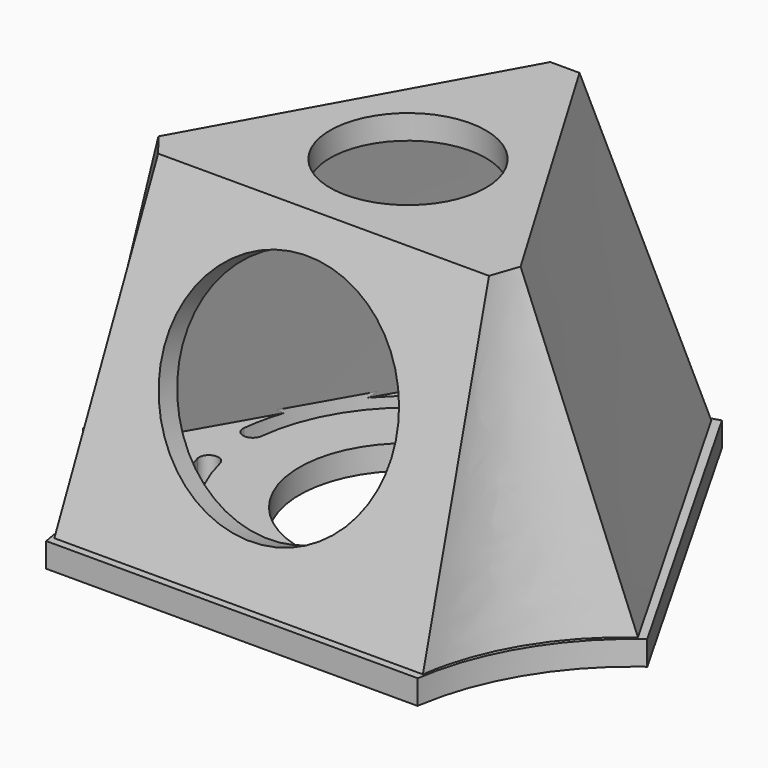
from build123d import *

# Parameters (mm, degrees)
F4_T      = -2.5
F6_R      = 8
F7_DEPTH  = 2.5
F9_DEPTH  = 2.5
F5_R      = 11.15
F10_DEPTH = 2.5
F12_DEPTH = 3
F14_R     = 12
F15_DEPTH = 2.5


with BuildPart() as f3:
    # F1 (on Top) → F3 section 0
    with BuildSketch(Plane.XY):
        with BuildLine():
            Line((-9.9467867985, 28.3880904317), (-28.9289951324, -4.7229221091))
            ThreePointArc((-28.9289951324, -4.7229221091), (-22.2240470788, -12.2883453364), (-19.0064776689, -21.8716226518))
            Line((-19.0064776689, -21.8716226518), (19.1736482084, -21.8716226518))
            ThreePointArc((19.1736482084, -21.8716226518), (22.5091585374, -12.4144453799), (29.3118748814, -5.0464821979))
            Line((29.3118748814, -5.0464821979), (10.2218100801, 28.3880904317))
            ThreePointArc((10.2218100801, 28.3880904317), (0.1375116408, 26.6367572465), (-9.9467867985, 28.3880904317))
        make_face()
    # F2 (on offset) → F3 section 1
    with BuildSketch(Plane.XY.offset(34)):
        Polygon((-1.6149276096, 21.1612877117), (-18.1069700896, -8.5710605783), (-16.2452941719, -10.9235407117), (17.7547058281, -10.9235407117), (18.7248919411, -8.0847489077), (1.3850723904, 21.1612877117), align=None)
    loft()

    # F4
    f4_openings = [f3.faces().sort_by_distance(p)[0] for p in [
        (0.146214, 0.67534, 0),
    ]]
    offset(amount=F4_T, openings=f4_openings)

    # F6 (on offset) → F7 (cut, through all)
    with BuildSketch(Plane.XY.offset(34)):
        with Locations((0, 0.8572275097)):
            Circle(F6_R)
    extrude(amount=-F7_DEPTH, mode=Mode.SUBTRACT)

    # F8 (on Top) → F9 (join)
    with BuildSketch(Plane.XY):
        with BuildLine():
            Line((-9.9509973079, 28.3981114626), (-28.9402902126, -4.7158375382))
            ThreePointArc((-28.9402902126, -4.7158375382), (-22.262978648, -12.2971961913), (-18.9997616398, -21.8583103269))
            Line((-18.9997616398, -21.8583103269), (19.1731229424, -21.8583103269))
            ThreePointArc((19.1731229424, -21.8583103269), (22.5411210843, -12.4278954037), (29.305677861, -5.044338759))
            Line((29.305677861, -5.044338759), (10.2393915877, 28.3862594515))
            ThreePointArc((10.2393915877, 28.3862594515), (0.1431471721, 26.6035220267), (-9.9509973079, 28.3981114626))
        make_face()
    extrude(amount=F9_DEPTH)

    # F5 (on Top) → F10 (cut, through all)
    with BuildSketch(Plane.XY):
        with Locations((0, 0.8448960521)):
            Circle(F5_R)
    extrude(amount=F10_DEPTH, mode=Mode.SUBTRACT)

    # F11 (on Top) → F12 (cut)
    with BuildSketch(Plane.XY):
        with BuildLine():
            ThreePointArc((-16.8968414401, 3.1769656869), (-12.6620659853, 12.6503778215), (-3.7095160029, 17.8973492754))
            ThreePointArc((-3.7095160029, 17.8973492754), (-2.9518202791, 19.0914586465), (-4.1459296503, 19.8491543702))
            ThreePointArc((-4.1459296503, 19.8491543702), (-14.1517208071, 13.9848921571), (-18.884705139, 3.3969609478))
            ThreePointArc((-18.884705139, 3.3969609478), (-18.00077092, 2.2930314679), (-16.8968414401, 3.1769656869))
        make_face()
        with BuildLine():
            ThreePointArc((-18.4914888461, -3.0593243269), (-12.8800677557, -12.6609521713), (-2.8559103373, -17.4771303206))
            ThreePointArc((-2.8559103373, -17.4771303206), (-1.7169605157, -16.6388026383), (-2.5552881974, -15.4998528163))
            ThreePointArc((-2.5552881974, -15.4998528163), (-11.5242711478, -11.19064079), (-16.5450163345, -2.5997106178))
            ThreePointArc((-16.5450163345, -2.5997106178), (-17.7480594441, -1.8562812201), (-18.4914888461, -3.0593243269))
        make_face()
        with BuildLine():
            ThreePointArc((16.5853291095, -2.4248646516), (11.6623008727, -11.0619365224), (2.7508780214, -15.4689491487))
            ThreePointArc((2.7508780214, -15.4689491487), (1.9258734863, -16.6175863922), (3.0745107298, -17.4425909273))
            ThreePointArc((3.0745107298, -17.4425909273), (13.0343362802, -12.5171062171), (18.5365443054, -2.8639082251))
            ThreePointArc((18.5365443054, -2.8639082251), (17.780458491, -1.6687788549), (16.5853291095, -2.4248646516))
        make_face()
        with BuildLine():
            ThreePointArc((4.3395190826, 17.7438114412), (12.8080809556, 12.4852465387), (16.8727439593, 3.383183053))
            ThreePointArc((16.8727439593, 3.383183053), (17.9873863481, 2.5127967631), (18.8577726667, 3.6274391295))
            ThreePointArc((18.8577726667, 3.6274391295), (14.3149139437, 13.8003337396), (4.850050497, 19.6775533254))
            ThreePointArc((4.850050497, 19.6775533254), (3.6279139689, 18.9659480585), (4.3395190826, 17.7438114412))
        make_face()
    extrude(amount=F12_DEPTH, mode=Mode.SUBTRACT)

    # F14 (on face) → F15 (cut, through all)
    with BuildSketch(Plane(origin=(0, -19.8168967703, 6.3810885188), x_dir=(1, 0, 0), z_dir=(0, -0.9518693028, 0.3065042095))):
        with Locations((0, 13.3294966072)):
            Circle(F14_R)
    extrude(amount=-F15_DEPTH, mode=Mode.SUBTRACT)


solid = f3.part
